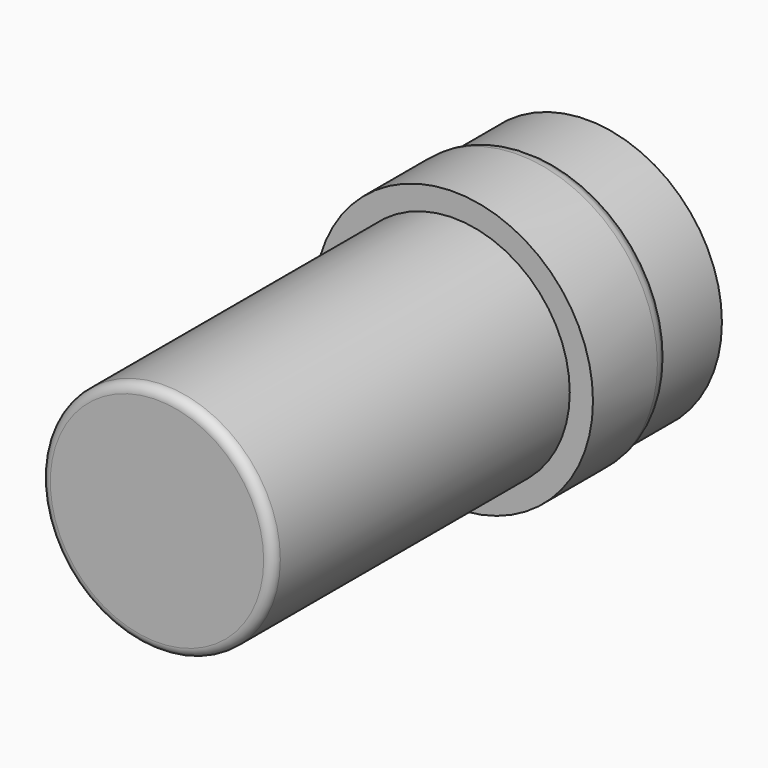
from build123d import *

# Parameters (mm, degrees)
F0_R     = 15
F1_DEPTH = 10
F2_R     = 12.5
F3_DEPTH = 40
F4_R     = 1
F5_R     = 14.5
F6_DEPTH = 8


# Not quite as in the source:
# - a fillet or chamfer that OpenCascade refuses, or shapes differently, is made with other operations: its cross-section is extruded or revolved along the edge and cut away or added


with BuildPart() as f1:
    # F0 (on Front) → F1 (new body)
    with BuildSketch(Plane.XZ):
        with Locations((-53.2553978264, 6.2320148572)):
            Circle(F0_R)
    extrude(amount=F1_DEPTH)

    # F2 (on face) → F3 (join)
    with BuildSketch(Plane.XZ.offset(10)):
        with Locations((-53.2553978264, 6.2320148572)):
            Circle(F2_R)
    extrude(amount=F3_DEPTH)

    # F4
    f4_edges = [f1.edges().sort_by_distance(p)[0] for p in [
        (-65.755398, -50, 6.232015),
    ]]
    fillet(f4_edges, radius=F4_R)

    # F5 (on face) → F6 (join)
    with BuildSketch(Plane(origin=(0, 0, 0), x_dir=(-1, 0, 0), z_dir=(0, 1, 0))):
        with Locations((53.2553978264, 6.2320148572)):
            Circle(F5_R)
    extrude(amount=F6_DEPTH)

    # F7: fillet of radius 2 on 1 edges, made by hand

    # F7_s1 → F7_t2 (revolve, cut)
    with BuildSketch(Plane.XY.offset(6.2320148572)):
        with BuildLine():
            ThreePointArc((-38.2553978264, -1.3228756555), (-38.384569133, -0.6157688743), (-38.7553978264, 0))
            Line((-38.7553978264, 0), (-38.2553978264, 0))
            Line((-38.2553978264, 0), (-38.2553978264, -1.3228756555))
        make_face()
    revolve(axis=Axis((-53.2553978264, 0, 6.2320148572), (0, -1, 0)), mode=Mode.SUBTRACT)


solid = f1.part
